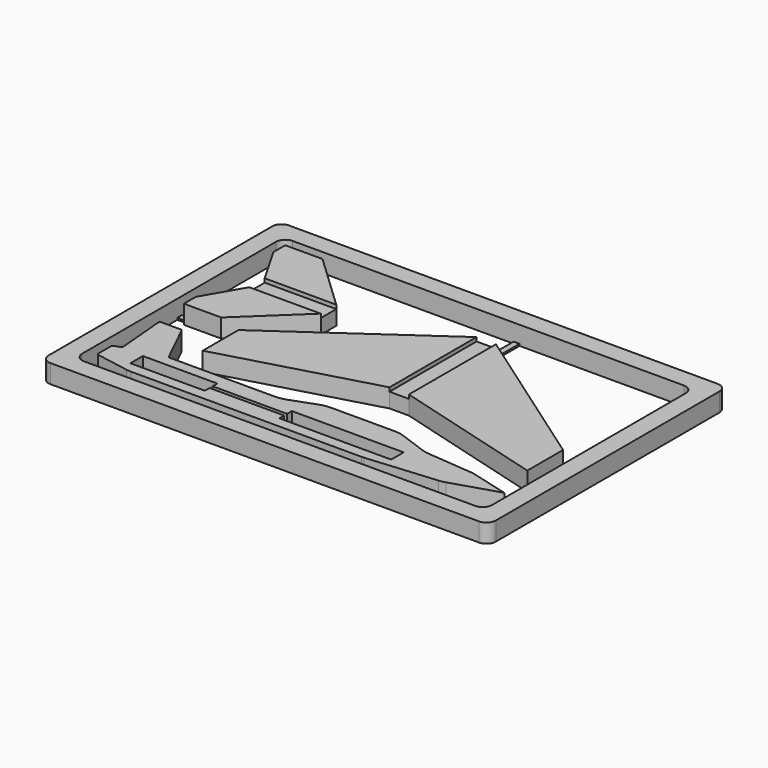
from build123d import *

# Parameters (mm, degrees)
F1_DEPTH    = 3.175
F3_DEPTH    = 3.175
F4_T1_DEPTH = 3.175
F4_T3_DEPTH = 5.3972120536
F4_T5_DEPTH = 7.65370531
F4_T7_DEPTH = 5.937328176
F4_T9_DEPTH = 4.2839879499
F5_R        = 0.3175
F7_DEPTH    = 25.4
F8_W        = 12.192
F8_H        = 3.302
F9_DEPTH    = 3.175
F10_W       = 12.192
F10_H       = 3.302
F11_DEPTH   = 0.6604
F12_W       = 3.302
F12_H       = 18.542
F13_DEPTH   = 3.175
F14_W       = 3.302
F14_H       = 18.542
F15_DEPTH   = 0.6604
F16_W       = 3.81
F16_H       = 1.016
F17_DEPTH   = 0.3175
F16_W_2     = 1.016
F16_H_2     = 7.62
F16_H_3     = 2.54
F16_W_3     = 2.54
F16_H_4     = 2.794


# Not quite as in the source:
# - a fillet or chamfer that OpenCascade refuses, or shapes differently, is made with other operations: its cross-section is extruded or revolved along the edge and cut away or added


with BuildPart() as f1:
    # F0 (on Top) → F1 (new body)
    with BuildSketch(Plane.XY):
        with BuildLine():
            ThreePointArc((0, 1.5875), (0.4649679849, 0.4649679849), (1.5875, 0))
            Line((1.5875, 0), (74.6125, 0))
            ThreePointArc((74.6125, 0), (75.7350320151, 0.4649679849), (76.2, 1.5875))
            Line((76.2, 1.5875), (76.2, 49.2125))
            ThreePointArc((76.2, 49.2125), (75.7350320151, 50.3350320151), (74.6125, 50.8))
            Line((74.6125, 50.8), (1.5875, 50.8))
            ThreePointArc((1.5875, 50.8), (0.4649679849, 50.3350320151), (0, 49.2125))
            Line((0, 49.2125), (0, 1.5875))
        make_face()
        with BuildLine():
            Line((73.025, 46.0375), (73.025, 4.7625))
            ThreePointArc((73.025, 4.7625), (72.5600320151, 3.6399679849), (71.4375, 3.175))
            Line((71.4375, 3.175), (4.7625, 3.175))
            ThreePointArc((4.7625, 3.175), (3.6399679849, 3.6399679849), (3.175, 4.7625))
            Line((3.175, 4.7625), (3.175, 46.0375))
            ThreePointArc((3.175, 46.0375), (3.6399679849, 47.1600320151), (4.7625, 47.625))
            Line((4.7625, 47.625), (71.4375, 47.625))
            ThreePointArc((71.4375, 47.625), (72.5600320151, 47.1600320151), (73.025, 46.0375))
        make_face(mode=Mode.SUBTRACT)
    extrude(amount=F1_DEPTH)


with BuildPart() as f3:
    # F2 (on Top) → F3 (new body)
    with BuildSketch(Plane.XY):
        Polygon((4.826, 5.8651659282), (11.0795292316, 4.7625), (50.9575292316, 4.7625), (63.6092018974, 5.8693779329), (72.0917764651, 8.5298344169), (65.3447845685, 10.337685447), (56.4886137024, 11.1125), (50.5215655604, 13.2843279101), (37.8215655604, 13.2843279101), (31.8545174184, 11.1125), (12.8045174184, 11.1125), (9.2493856396, 18.4016003435), (5.4393856396, 18.4016003435), (6.2142001926, 9.5454294775), (4.826, 9.0401659282), align=None)
    extrude(amount=F3_DEPTH)

    # F4: fillet of radius 5.08 on 8 edges, made by hand

    # F4_s2 → F4_t1 (join)
    with BuildSketch(Plane.XY):
        with BuildLine():
            ThreePointArc((57.1548634245, 11.0542107022), (56.4981013588, 11.1552960524), (55.8601522695, 11.341241255))
            Line((55.8601522695, 11.341241255), (56.4886137024, 11.1125))
            Line((56.4886137024, 11.1125), (57.1548634245, 11.0542107022))
        make_face()
        with BuildLine():
            ThreePointArc((32.6962386845, 11.4188614864), (31.840909099, 11.1896766147), (30.9587763564, 11.1125))
            Line((30.9587763564, 11.1125), (31.8545174184, 11.1125))
            Line((31.8545174184, 11.1125), (32.6962386845, 11.4188614864))
        make_face()
    extrude(amount=F4_T1_DEPTH)

    # F4_s4 → F4_t3 (cut)
    with BuildSketch(Plane.XY.offset(-1.1111060268)):
        with BuildLine():
            ThreePointArc((65.7740829713, 10.2226552866), (65.3414149647, 10.3185754744), (64.9020333953, 10.3764211554))
            Line((64.9020333953, 10.3764211554), (65.3447845685, 10.337685447))
            Line((65.3447845685, 10.337685447), (65.7740829713, 10.2226552866))
        make_face()
        with BuildLine():
            ThreePointArc((10.6418388998, 4.8396766147), (11.0812204692, 4.7818309337), (11.5239716423, 4.7625))
            Line((11.5239716423, 4.7625), (11.0795292316, 4.7625))
            Line((11.0795292316, 4.7625), (10.6418388998, 4.8396766147))
        make_face()
    extrude(amount=F4_T3_DEPTH, mode=Mode.SUBTRACT)

    # F4_s6 → F4_t5 (cut)
    with BuildSketch(Plane.XY.offset(-2.239352655)):
        with BuildLine():
            ThreePointArc((51.3632868265, 12.9779664237), (50.507957241, 13.2071512954), (49.6258244984, 13.2843279101))
            Line((49.6258244984, 13.2843279101), (50.5215655604, 13.2843279101))
            Line((50.5215655604, 13.2843279101), (51.3632868265, 12.9779664237))
        make_face()
        with BuildLine():
            ThreePointArc((38.7173066224, 13.2843279101), (37.8351738799, 13.2071512954), (36.9798442943, 12.9779664237))
            Line((36.9798442943, 12.9779664237), (37.8215655604, 13.2843279101))
            Line((37.8215655604, 13.2843279101), (38.7173066224, 13.2843279101))
        make_face()
    extrude(amount=F4_T5_DEPTH, mode=Mode.SUBTRACT)

    # F4_s8 → F4_t7 (cut)
    with BuildSketch(Plane.XY.offset(-1.381164088)):
        with BuildLine():
            ThreePointArc((63.0588385607, 5.8212273801), (63.6033805865, 5.8987596693), (64.1363482356, 6.0347109792))
            Line((64.1363482356, 6.0347109792), (63.6092018974, 5.8693779329))
            Line((63.6092018974, 5.8693779329), (63.0588385607, 5.8212273801))
        make_face()
    extrude(amount=F4_T7_DEPTH, mode=Mode.SUBTRACT)

    # F4_s10 → F4_t9 (cut)
    with BuildSketch(Plane.XY.offset(-0.5544939749)):
        with BuildLine():
            ThreePointArc((50.7357316417, 4.7625), (50.9573181295, 4.7673350344), (51.1784828148, 4.7818309337))
            Line((51.1784828148, 4.7818309337), (50.9575292316, 4.7625))
            Line((50.9575292316, 4.7625), (50.7357316417, 4.7625))
        make_face()
    extrude(amount=F4_T9_DEPTH, mode=Mode.SUBTRACT)

    # F5
    f5_edges = [f3.edges().sort_by_distance(p)[0] for p in [
        (4.826, 5.865166, 1.5875),
        (4.826, 9.040166, 1.5875),
        (6.2142, 9.545429, 1.5875),
        (5.439386, 18.4016, 1.5875),
        (9.249386, 18.4016, 1.5875),
        (12.804517, 11.1125, 1.5875),
    ]]
    fillet(f5_edges, radius=F5_R)

    # F6 (on face) → F7 (cut)
    with BuildSketch(Plane.XY.offset(3.175)):
        Polygon((22.606, 9.271), (9.906, 9.271), (9.906, 6.604), (22.606, 6.604), (22.606, 7.62), (35.306, 7.62), (35.306, 6.604), (54.356, 6.604), (54.356, 9.271), (35.306, 9.271), (35.306, 8.255), (22.606, 8.255), align=None)
    extrude(amount=-F7_DEPTH, mode=Mode.SUBTRACT)


with BuildPart() as f9:
    # F8 (on Top) → F9 (new body)
    with BuildSketch(Plane.XY):
        Polygon((4.7625, 43.4975), (8.5725, 36.8983864232), (20.7645, 36.8983864232), (11.1125, 46.0375), (4.7625, 46.0375), align=None)
        with Locations((14.6685, 35.2473864232)):
            Rectangle(F8_W, F8_H)
        Polygon((20.7645, 33.5963864232), (8.5725, 33.5963864232), (4.7625, 26.9972728463), (4.7625, 24.4572728463), (11.1125, 24.4572728463), align=None)
    extrude(amount=F9_DEPTH)

    # F10 (on face) → F11 (cut)
    with BuildSketch(Plane.XY.offset(3.175)):
        with Locations((14.6685, 35.2473864232)):
            Rectangle(F10_W, F10_H)
    extrude(amount=-F11_DEPTH, mode=Mode.SUBTRACT)


with BuildPart() as f13:
    # F12 (on Top) → F13 (new body)
    with BuildSketch(Plane.XY):
        with Locations((42.8259225938, 32.004)):
            Rectangle(F12_W, F12_H)
        Polygon((41.1749225938, 22.733), (41.1749225938, 41.275), (15.1668451876, 23.0639481459), (15.1668451876, 15.4439481459), align=None)
        Polygon((70.485, 23.0639481459), (44.4769225938, 41.275), (44.4769225938, 22.733), (70.485, 15.4439481459), align=None)
    extrude(amount=F13_DEPTH)

    # F14 (on face) → F15 (cut)
    with BuildSketch(Plane.XY.offset(3.175)):
        with Locations((42.8259225938, 32.004)):
            Rectangle(F14_W, F14_H)
    extrude(amount=-F15_DEPTH, mode=Mode.SUBTRACT)


with BuildPart() as f17:
    # F16 (on Top) → F17 (new body)
    with BuildSketch(Plane.XY):
        with Locations((71.755, 18.923)):
            Rectangle(F16_W, F16_H)
    extrude(amount=F17_DEPTH)


with BuildPart() as f17b:
    # F16 (on Top) → F17, piece 2 (new body)
    with BuildSketch(Plane.XY):
        with Locations((42.9211696643, 44.4056276325)):
            Rectangle(F16_W_2, F16_H_2)
    extrude(amount=F17_DEPTH)


with BuildPart() as f17c:
    # F16 (on Top) → F17, piece 3 (new body)
    with BuildSketch(Plane.XY):
        with Locations((47.117, 3.81)):
            Rectangle(F16_W_2, F16_H_3)
    extrude(amount=F17_DEPTH)


with BuildPart() as f17d:
    # F16 (on Top) → F17, piece 4 (new body)
    with BuildSketch(Plane.XY):
        with Locations((16.383, 3.81)):
            Rectangle(F16_W_2, F16_H_3)
    extrude(amount=F17_DEPTH)


with BuildPart() as f17e:
    # F16 (on Top) → F17, piece 5 (new body)
    with BuildSketch(Plane.XY):
        with Locations((3.81, 25.527)):
            Rectangle(F16_W_3, F16_H)
    extrude(amount=F17_DEPTH)


with BuildPart() as f17f:
    # F16 (on Top) → F17, piece 6 (new body)
    with BuildSketch(Plane.XY):
        with Locations((7.493, 46.863)):
            Rectangle(F16_W_2, F16_H_4)
    extrude(amount=F17_DEPTH)


solid = Compound([f1.part, f3.part, f9.part, f13.part, f17.part, f17b.part, f17c.part, f17d.part, f17e.part, f17f.part])
